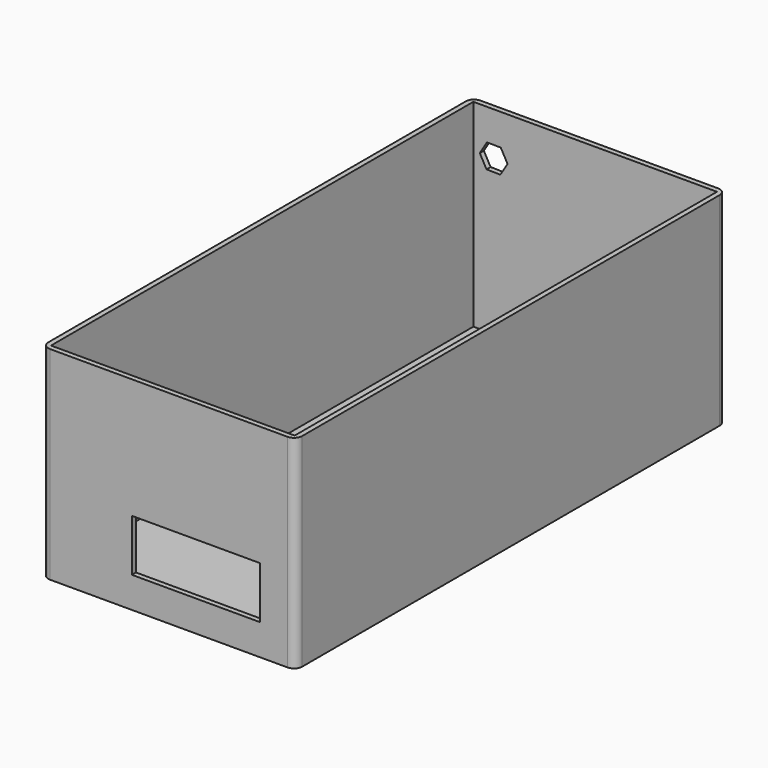
from build123d import *

# Parameters (mm, degrees)
F0_W            = 63.5
F0_H            = 50.8
F1_DEPTH        = 134.62
F2_T            = -1.27
F3_W            = 32
F3_H            = 13
F4_DEPTH        = 25.4
F6_R            = 1.6
F7_DEPTH        = 25.4
F7_COPIES_COUNT = 2
F7_COPIES_PITCH = 90.921425
F8_R            = 2.032
F9_R            = 2.032
F10_R           = 2.032
F11_DEPTH       = 25.4


# Not quite as in the source:
# - a pattern or mirror of a feature is missing from the dataset's text; its kind, count and spacing are read off the source's solid
# - a feature names something its author has since deleted; it is built from what else it names


with BuildPart() as f1:
    # F0 (on Front) → F1 (new body)
    with BuildSketch(Plane.XZ):
        Rectangle(F0_W, F0_H)
    extrude(amount=F1_DEPTH)

    # F2
    f2_openings = [f1.faces().sort_by_distance(p)[0] for p in [
        (0, -67.31, 25.4),
    ]]
    offset(amount=F2_T, openings=f2_openings)

    # F3 (on face) → F4 (cut)
    with BuildSketch(Plane.XZ.offset(134.62)):
        with Locations((6.7759254016, -11.1641568676)):
            Rectangle(F3_W, F3_H)
    extrude(amount=-F4_DEPTH, mode=Mode.SUBTRACT)

    # F6 (on face) → F7 (cut)
    with BuildSketch(Plane.XY.offset(-24.13)):
        with Locations((-22.3445058558, -16.729145626)):
            Circle(F6_R)
        with Locations((-22.3445058558, -91.629145626)):
            Circle(F6_R)
        with Locations((25.4725906998, -97.8303775191)):
            Circle(F6_R)
    f7 = extrude(amount=-F7_DEPTH, mode=Mode.SUBTRACT)

    # F7_copies: F7 ×2
    with Locations(*[Vector(0.5370160888, 0.8435720007, 0) * (i * F7_COPIES_PITCH) for i in range(1, F7_COPIES_COUNT)]):
        add(f7, mode=Mode.SUBTRACT)

    # F8
    f8_edges = [f1.edges().sort_by_distance(p)[0] for p in [
        (-31.75, -134.62, 0),
    ]]
    fillet(f8_edges, radius=F8_R)

    # F9
    f9_edges = [f1.edges().sort_by_distance(p)[0] for p in [
        (31.75, -134.62, 0),
    ]]
    fillet(f9_edges, radius=F9_R)

    # F10
    f10_edges = [f1.edges().sort_by_distance(p)[0] for p in [
        (31.75, 0, 0),
        (-31.75, 0, 0),
    ]]
    fillet(f10_edges, radius=F10_R)

    # F5 (on face) → F11 (cut)
    with BuildSketch(Plane(origin=(0, 0, 0), x_dir=(-1, 0, 0), z_dir=(0, 1, 0))):
        Polygon((-21.936369905, 14.6150602972), (-23.7176816564, 17.5860750134), (-27.1813117514, 17.5289211427), (-28.863630095, 14.5007525558), (-27.0823183436, 11.5297378396), (-23.6186882486, 11.5868917102), align=None)
        Polygon((21.936369905, 14.5007525558), (23.7176816564, 11.5297378396), (27.1813117514, 11.5868917102), (28.863630095, 14.6150602972), (27.0823183436, 17.5860750134), (23.6186882486, 17.5289211427), align=None)
    extrude(amount=-F11_DEPTH, mode=Mode.SUBTRACT)


solid = f1.part
